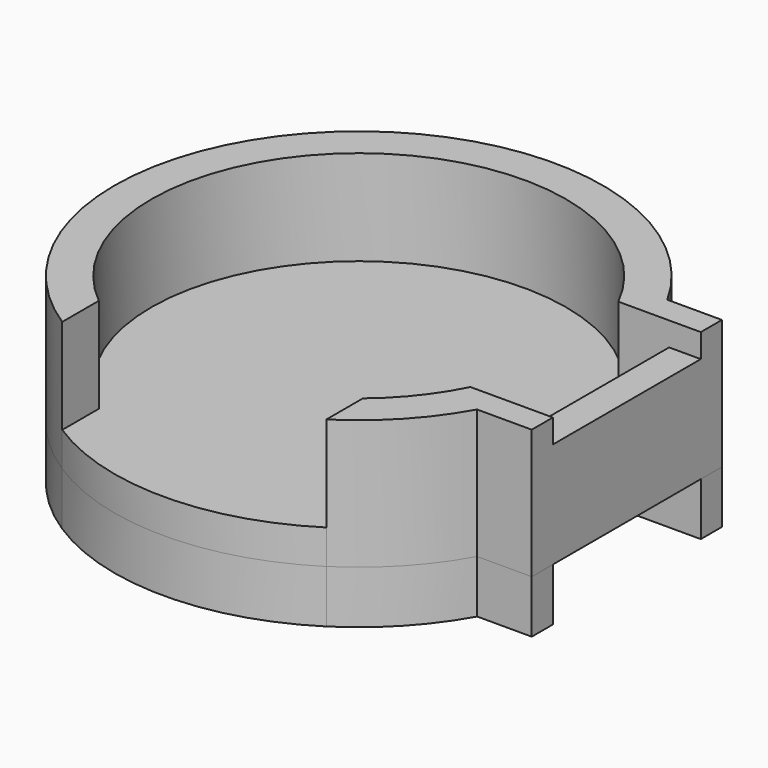
from build123d import *

# Parameters (mm, degrees)
F0_W     = 1.2
F0_H     = 7
F1_DEPTH = 1.3
F2_DEPTH = 4.9
F3_DEPTH = 4
F4_DEPTH = 2


with BuildPart() as f1:
    # F0 (on Top) → F1 (new body)
    with BuildSketch(Plane.XY):
        with BuildLine():
            ThreePointArc((-5, -6.0516526668), (-4.8821358287, 6.147133458), (7.026556767, 3.5))
            Line((7.026556767, 3.5), (8.95, 3.5))
            Line((8.95, 3.5), (10.15, 3.5))
            Line((10.15, 3.5), (10.15, 4.5))
            Line((10.15, 4.5), (8.0816149376, 4.5))
            ThreePointArc((8.0816149376, 4.5), (-6.3314408213, 6.7435418828), (-5, -7.7821912081))
            Line((-5, -7.7821912081), (-5, -6.0516526668))
        make_face()
        with BuildLine():
            ThreePointArc((5, -6.0516526668), (0, -7.85), (-5, -6.0516526668))
            Line((-5, -6.0516526668), (-5, -7.7821912081))
            ThreePointArc((-5, -7.7821912081), (0, -9.25), (5, -7.7821912081))
            Line((5, -7.7821912081), (5, -6.0516526668))
        make_face()
        with Locations((9.55, 0)):
            Rectangle(F0_W, F0_H)
        with BuildLine():
            ThreePointArc((7.026556767, -3.5), (6.147133458, -4.8821358287), (5, -6.0516526668))
            Line((5, -6.0516526668), (5, -7.7821912081))
            ThreePointArc((5, -7.7821912081), (6.7435418828, -6.3314408213), (8.0816149376, -4.5))
            Line((8.0816149376, -4.5), (10.15, -4.5))
            Line((10.15, -4.5), (10.15, -3.5))
            Line((10.15, -3.5), (8.95, -3.5))
            Line((8.95, -3.5), (7.026556767, -3.5))
        make_face()
        with BuildLine():
            Line((8.95, 3.5), (7.026556767, 3.5))
            Line((7.026556767, 3.5), (6.75, 3.5))
            Line((6.75, 3.5), (6.0621778265, 3.5))
            ThreePointArc((6.0621778265, 3.5), (6.761480784, 1.8117333157), (7, 0))
            ThreePointArc((7, 0), (6.761480784, -1.8117333157), (6.0621778265, -3.5))
            Line((6.0621778265, -3.5), (6.75, -3.5))
            Line((6.75, -3.5), (7.026556767, -3.5))
            Line((7.026556767, -3.5), (8.95, -3.5))
            Line((8.95, -3.5), (8.95, 3.5))
        make_face()
        with BuildLine():
            ThreePointArc((7, 0), (6.761480784, 1.8117333157), (6.0621778265, 3.5))
            ThreePointArc((6.0621778265, 3.5), (-7, 0), (6.0621778265, -3.5))
            ThreePointArc((6.0621778265, -3.5), (6.761480784, -1.8117333157), (7, 0))
        make_face()
        with BuildLine():
            Line((6.75, 3.5), (7.026556767, 3.5))
            ThreePointArc((7.026556767, 3.5), (-4.8821358287, 6.147133458), (-5, -6.0516526668))
            ThreePointArc((-5, -6.0516526668), (0, -7.85), (5, -6.0516526668))
            ThreePointArc((5, -6.0516526668), (6.147133458, -4.8821358287), (7.026556767, -3.5))
            Line((7.026556767, -3.5), (6.75, -3.5))
            Line((6.75, -3.5), (6.0621778265, -3.5))
            ThreePointArc((6.0621778265, -3.5), (-7, 0), (6.0621778265, 3.5))
            Line((6.0621778265, 3.5), (6.75, 3.5))
        make_face()
    extrude(amount=F1_DEPTH)

    # F0 (on Top) → F2 (join)
    with BuildSketch(Plane.XY):
        with BuildLine():
            ThreePointArc((-5, -6.0516526668), (-4.8821358287, 6.147133458), (7.026556767, 3.5))
            Line((7.026556767, 3.5), (8.95, 3.5))
            Line((8.95, 3.5), (10.15, 3.5))
            Line((10.15, 3.5), (10.15, 4.5))
            Line((10.15, 4.5), (8.0816149376, 4.5))
            ThreePointArc((8.0816149376, 4.5), (-6.3314408213, 6.7435418828), (-5, -7.7821912081))
            Line((-5, -7.7821912081), (-5, -6.0516526668))
        make_face()
        with BuildLine():
            ThreePointArc((7.026556767, -3.5), (6.147133458, -4.8821358287), (5, -6.0516526668))
            Line((5, -6.0516526668), (5, -7.7821912081))
            ThreePointArc((5, -7.7821912081), (6.7435418828, -6.3314408213), (8.0816149376, -4.5))
            Line((8.0816149376, -4.5), (10.15, -4.5))
            Line((10.15, -4.5), (10.15, -3.5))
            Line((10.15, -3.5), (8.95, -3.5))
            Line((8.95, -3.5), (7.026556767, -3.5))
        make_face()
    extrude(amount=F2_DEPTH)

    # F0 (on Top) → F3 (join)
    with BuildSketch(Plane.XY):
        with Locations((9.55, 0)):
            Rectangle(F0_W, F0_H)
    extrude(amount=F3_DEPTH)


with BuildPart() as f4:
    # F0 (on Top) → F4 (new body)
    with BuildSketch(Plane.XY):
        with BuildLine():
            ThreePointArc((-5, -6.0516526668), (-4.8821358287, 6.147133458), (7.026556767, 3.5))
            Line((7.026556767, 3.5), (8.95, 3.5))
            Line((8.95, 3.5), (10.15, 3.5))
            Line((10.15, 3.5), (10.15, 4.5))
            Line((10.15, 4.5), (8.0816149376, 4.5))
            ThreePointArc((8.0816149376, 4.5), (-6.3314408213, 6.7435418828), (-5, -7.7821912081))
            Line((-5, -7.7821912081), (-5, -6.0516526668))
        make_face()
        with BuildLine():
            ThreePointArc((5, -6.0516526668), (0, -7.85), (-5, -6.0516526668))
            Line((-5, -6.0516526668), (-5, -7.7821912081))
            ThreePointArc((-5, -7.7821912081), (0, -9.25), (5, -7.7821912081))
            Line((5, -7.7821912081), (5, -6.0516526668))
        make_face()
        with BuildLine():
            ThreePointArc((7.026556767, -3.5), (6.147133458, -4.8821358287), (5, -6.0516526668))
            Line((5, -6.0516526668), (5, -7.7821912081))
            ThreePointArc((5, -7.7821912081), (6.7435418828, -6.3314408213), (8.0816149376, -4.5))
            Line((8.0816149376, -4.5), (10.15, -4.5))
            Line((10.15, -4.5), (10.15, -3.5))
            Line((10.15, -3.5), (8.95, -3.5))
            Line((8.95, -3.5), (7.026556767, -3.5))
        make_face()
        with BuildLine():
            Line((6.75, 3.5), (7.026556767, 3.5))
            ThreePointArc((7.026556767, 3.5), (-4.8821358287, 6.147133458), (-5, -6.0516526668))
            ThreePointArc((-5, -6.0516526668), (0, -7.85), (5, -6.0516526668))
            ThreePointArc((5, -6.0516526668), (6.147133458, -4.8821358287), (7.026556767, -3.5))
            Line((7.026556767, -3.5), (6.75, -3.5))
            Line((6.75, -3.5), (6.0621778265, -3.5))
            ThreePointArc((6.0621778265, -3.5), (-7, 0), (6.0621778265, 3.5))
            Line((6.0621778265, 3.5), (6.75, 3.5))
        make_face()
    extrude(amount=-F4_DEPTH)


solid = Compound([f1.part, f4.part])
